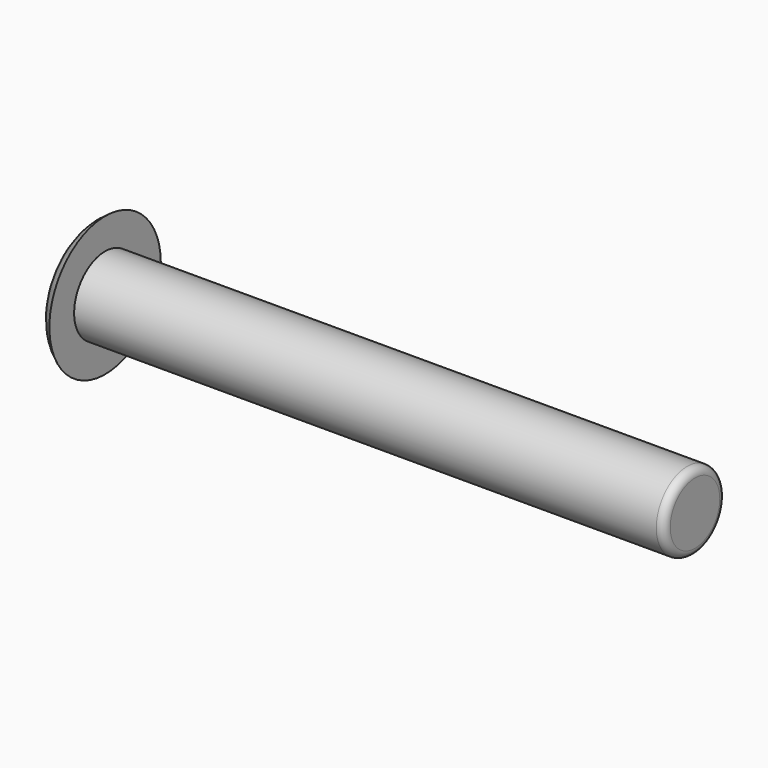
from build123d import *

# Parameters (mm, degrees)
F0_R     = 5
F2_DEPTH = 76.2
F1_R     = 9
F3_DEPTH = 2.5
F5_R     = 1


# Not quite as in the source:
# - a fillet or chamfer that OpenCascade refuses, or shapes differently, is made with other operations: its cross-section is extruded or revolved along the edge and cut away or added


with BuildPart() as f2:
    # F0 (on Right) → F2 (new body)
    with BuildSketch(Plane.YZ):
        Circle(F0_R)
    extrude(amount=F2_DEPTH)

    # F1 (on Right) → F3 (join)
    with BuildSketch(Plane.YZ):
        Circle(F1_R)
    extrude(amount=-F3_DEPTH)

    # F4: fillet of radius 5 on 1 edges, made by hand

    # F4_s1 → F4_t2 (revolve, cut)
    with BuildSketch(Plane.XY):
        with BuildLine():
            ThreePointArc((0, 9), (-1.8301270189, 7.1698729811), (-2.5, 4.6698729811))
            Line((-2.5, 4.6698729811), (-2.5, 9))
            Line((-2.5, 9), (0, 9))
        make_face()
    revolve(axis=Axis((-2.5, 0, 0), (1, 0, 0)), mode=Mode.SUBTRACT)

    # F5
    f5_edges = [f2.edges().sort_by_distance(p)[0] for p in [
        (76.2, -5, 0),
    ]]
    fillet(f5_edges, radius=F5_R)


solid = f2.part
